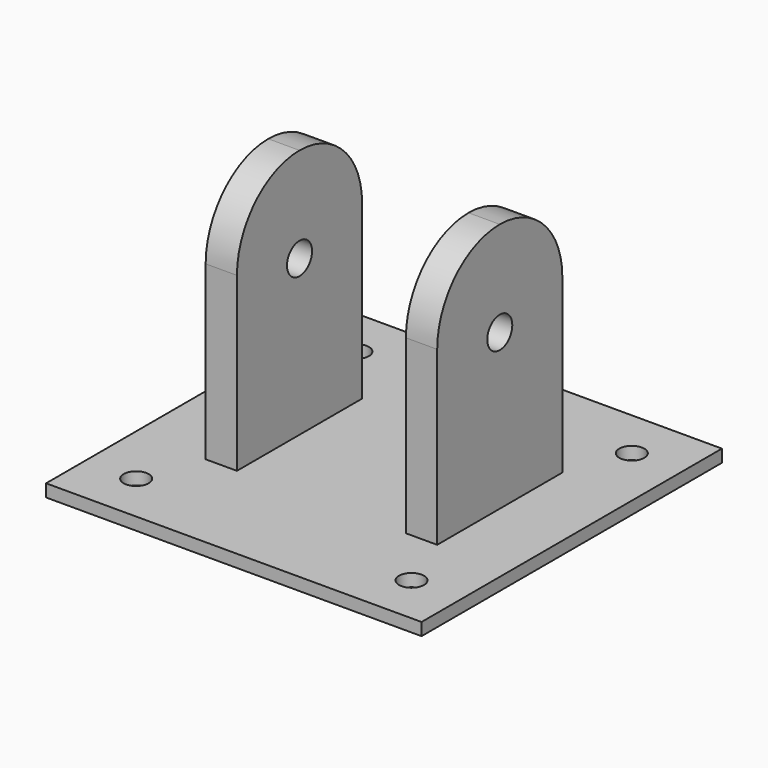
from build123d import *

# Parameters (mm, degrees)
F0_W     = 60
F0_H     = 60
F1_DEPTH = 2
F2_W     = 5
F2_H     = 25
F3_DEPTH = 40
F4_DEPTH = 40
F5_R     = 12.49999
F7_D     = 5
F9_D     = 4
F9_DEPTH = 15
F9_TIP   = 1.2017212381


# Not quite as in the source:
# - a fillet or chamfer is up to 0.001 mm smaller than in the source, because OpenCascade refuses the exact size


with BuildPart() as f1:
    # F0 (on Top) → F1 (new body)
    with BuildSketch(Plane.XY):
        with Locations((35.6504749941, -30)):
            Rectangle(F0_W, F0_H)
    extrude(amount=F1_DEPTH)

    # F2 (on face) → F3 (join)
    with BuildSketch(Plane.XY.offset(2)):
        with Locations((19.6504749941, -30)):
            Rectangle(F2_W, F2_H)
    extrude(amount=F3_DEPTH)

    # F2 (on face) → F4 (join)
    with BuildSketch(Plane.XY.offset(2)):
        with Locations((51.6504749941, -30)):
            Rectangle(F2_W, F2_H)
    extrude(amount=F4_DEPTH)

    # F5 (radius 12.5 in the source; OpenCascade refuses exactly that, so slightly less here)
    f5_edges = [f1.edges().sort_by_distance(p)[0] for p in [
        (19.650475, -42.5, 42),
        (51.650475, -42.5, 42),
        (51.650475, -17.5, 42),
        (19.650475, -17.5, 42),
    ]]
    fillet(f5_edges, radius=F5_R)

    # F7 (through all)
    with Locations(Plane(origin=(17.1504749941, 0, 0), x_dir=(0, -1, 0), z_dir=(-1, 0, 0))):
        with Locations((30, 26.8072411418)):
            Hole(F7_D / 2)

    # F9
    with Locations(Plane.XY.offset(2)):
        with Locations((13.6504749941, -8), (13.6504749941, -52), (57.6504749941, -52), (57.6504749941, -8)):
            Hole(F9_D / 2, depth=F9_DEPTH)
            with Locations((0, 0, -(F9_DEPTH + F9_TIP / 2))):  # 118° drill point
                Cone(0, F9_D / 2, F9_TIP, mode=Mode.SUBTRACT)


solid = f1.part
